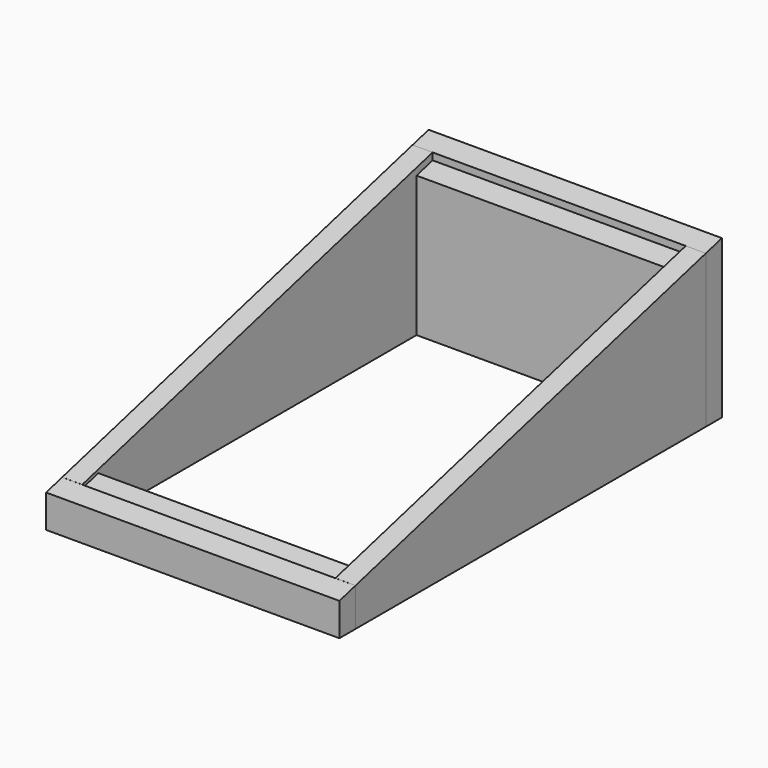
from build123d import *

# Parameters (mm, degrees)
F1_DEPTH   = 36.255
F2_DEPTH   = 39.3
F3_DEPTH   = 9.5
F4_DEPTH   = 10
F5_DEPTH   = 38
F6_SIZE2   = 28.489896
F6_SIZE    = 108.99999
F7_SIZE2   = 1.306866
F7_SIZE    = 4.99999
F7_2_SIZE2 = 1.306866
F7_2_SIZE  = 4.99999
F8_SIZE2   = 1.306866
F8_SIZE    = 4.99999
F8_2_SIZE2 = 1.306866
F8_2_SIZE  = 4.99999
F9_SIZE2   = 28.489896
F9_SIZE    = 108.99999


# Not quite as in the source:
# - a fillet or chamfer is up to 0.001 mm smaller than in the source, because OpenCascade refuses the exact size


with BuildPart() as f1:
    # F0 (on Top) → F1 (new body)
    with BuildSketch(Plane.XY):
        Polygon((63, -5), (63, 0), (0, 0), (0, -5), (5, -5), (58, -5), align=None)
    extrude(amount=F1_DEPTH)

    # F0 (on Top) → F2 (join)
    with BuildSketch(Plane.XY):
        Polygon((0, 0), (63, 0), (68, 0), (68, 5), (-5, 5), (-5, 0), align=None)
    extrude(amount=F2_DEPTH)

    # F7#2 (size 5 and 1.3068764239 in the source; OpenCascade refuses exactly that, so slightly less here)
    f7_2_edges = [f1.edges().sort_by_distance(p)[0] for p in [
        (31.5, 0, 39.3),
    ]]
    f7_2_side = f1.faces().sort_by_distance((31.5, 2.5, 39.3))[0]
    chamfer(f7_2_edges, length=F7_2_SIZE, length2=F7_2_SIZE2, reference=f7_2_side)

    # F8 (size 5 and 1.3068764239 in the source; OpenCascade refuses exactly that, so slightly less here)
    f8_edges = [f1.edges().sort_by_distance(p)[0] for p in [
        (31.5, -5, 36.255),
    ]]
    f8_side = f1.faces().sort_by_distance((31.5, -2.5, 36.255))[0]
    chamfer(f8_edges, length=F8_SIZE, length2=F8_SIZE2, reference=f8_side)


with BuildPart() as f3:
    # F0 (on Top) → F3 (new body)
    with BuildSketch(Plane.XY):
        Polygon((68, -114), (68, -109), (63, -109), (0, -109), (-5, -109), (-5, -114), align=None)
    extrude(amount=F3_DEPTH)

    # F7 (size 5 and 1.3068764239 in the source; OpenCascade refuses exactly that, so slightly less here)
    f7_edges = [f3.edges().sort_by_distance(p)[0] for p in [
        (31.5, -114, 9.5),
    ]]
    f7_side = f3.faces().sort_by_distance((31.5, -111.5, 9.5))[0]
    chamfer(f7_edges, length=F7_SIZE, length2=F7_SIZE2, reference=f7_side)


with BuildPart() as f4:
    # F0 (on Top) → F4 (new body)
    with BuildSketch(Plane.XY):
        Polygon((63, -109), (63, -104), (58, -104), (5, -104), (0, -104), (0, -109), align=None)
    extrude(amount=F4_DEPTH)

    # F8#2 (size 5 and 1.3068764239 in the source; OpenCascade refuses exactly that, so slightly less here)
    f8_2_edges = [f4.edges().sort_by_distance(p)[0] for p in [
        (31.5, -109, 10),
    ]]
    f8_2_side = f4.faces().sort_by_distance((31.5, -106.5, 10))[0]
    chamfer(f8_2_edges, length=F8_2_SIZE, length2=F8_2_SIZE2, reference=f8_2_side)


with BuildPart() as f5:
    # F0 (on Top) → F5 (new body)
    with BuildSketch(Plane.XY):
        Polygon((68, 0), (63, 0), (63, -5), (63, -104), (63, -109), (68, -109), align=None)
    extrude(amount=F5_DEPTH)

    # F6 (size 109 and 28.4899060414 in the source; OpenCascade refuses exactly that, so slightly less here)
    f6_edges = [f5.edges().sort_by_distance(p)[0] for p in [
        (65.5, -109, 38),
    ]]
    f6_side = f5.faces().sort_by_distance((65.5, -54.5, 38))[0]
    chamfer(f6_edges, length=F6_SIZE, length2=F6_SIZE2, reference=f6_side)


with BuildPart() as f5b:
    # F0 (on Top) → F5, piece 2 (new body)
    with BuildSketch(Plane.XY):
        Polygon((0, -5), (0, 0), (-5, 0), (-5, -109), (0, -109), (0, -104), align=None)
    extrude(amount=F5_DEPTH)

    # F9 (size 109 and 28.4899060414 in the source; OpenCascade refuses exactly that, so slightly less here)
    f9_edges = [f5b.edges().sort_by_distance(p)[0] for p in [
        (-2.5, -109, 38),
    ]]
    f9_side = f5b.faces().sort_by_distance((-2.5, -54.5, 38))[0]
    chamfer(f9_edges, length=F9_SIZE, length2=F9_SIZE2, reference=f9_side)


solid = Compound([f1.part, f3.part, f4.part, f5.part, f5b.part])
